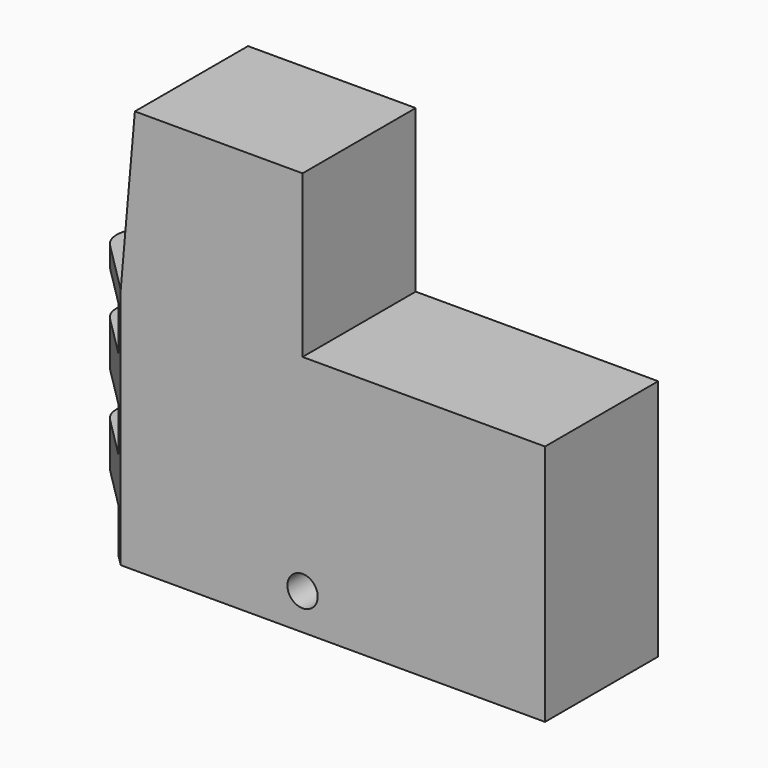
from build123d import *

# Parameters (mm, degrees)
F0_W       = 152.4
F0_H       = 76.2
F1_DEPTH   = 44.45
F2_W       = 15.24
F2_H       = 13.97
F3_DEPTH   = 44.451
F4_R       = 3.175
F5_DEPTH   = 69.85
F6_C1_SIZE = 19.05
F6_C2_SIZE = 19.05
F7_R       = 4.7625
F8_DEPTH   = 44.451
F10_DEPTH  = 44.45
F11_R      = 7.62


with BuildPart() as f1:
    # F0 (on Front) → F1 (new body)
    with BuildSketch(Plane.XZ):
        with Locations((76.2, 38.1)):
            Rectangle(F0_W, F0_H)
    extrude(amount=F1_DEPTH)

    # F2 (on face) → F3 (cut, through all)
    with BuildSketch(Plane.XZ.offset(44.45)):
        with Locations((7.62, 6.985)):
            Rectangle(F2_W, F2_H)
        with Locations((7.62, 34.925)):
            Rectangle(F2_W, F2_H)
        with Locations((7.62, 62.865)):
            Rectangle(F2_W, F2_H)
    extrude(amount=-F3_DEPTH, mode=Mode.SUBTRACT)

    # F4 (on face) → F5 (cut)
    with BuildSketch(Plane(origin=(0, 0, 0), x_dir=(1, 0, 0), z_dir=(0, 0, -1))):
        with Locations((6.35, 22.225)):
            Circle(F4_R)
    extrude(amount=-F5_DEPTH, mode=Mode.SUBTRACT)

    # F6: chamfer of 19.05 on 6 edges, made by hand

    # F6_c1
    f6_c1_edges = [f1.edges().sort_by_distance(p)[0] for p in [
        (0, 0, 73.025),
    ]]
    chamfer(f6_c1_edges, length=F6_C1_SIZE)

    # F6_c2
    f6_c2_edges = [f1.edges().sort_by_distance(p)[0] for p in [
        (0, -44.45, 73.025),
    ]]
    chamfer(f6_c2_edges, length=F6_C2_SIZE)

    # F7 (on face) → F8 (cut, through all)
    with BuildSketch(Plane.XZ.offset(44.45)):
        with Locations((76.2, 11.43)):
            Circle(F7_R)
    extrude(amount=-F8_DEPTH, mode=Mode.SUBTRACT)

    # F9 (on face) → F10 (join)
    with BuildSketch(Plane.XZ.offset(44.45)):
        Polygon((23.4944241071, 127), (19.05, 76.2), (76.2, 76.2), (76.2, 127), align=None)
    extrude(amount=-F10_DEPTH)

    # F11
    f11_edges = [f1.edges().sort_by_distance(p)[0] for p in [
        (0, -19.05, 73.025),
        (0, -25.4, 73.025),
        (0, -25.4, 48.895),
        (0, -19.05, 48.895),
        (0, -19.05, 20.955),
        (0, -25.4, 20.955),
    ]]
    fillet(f11_edges, radius=F11_R)


solid = f1.part
